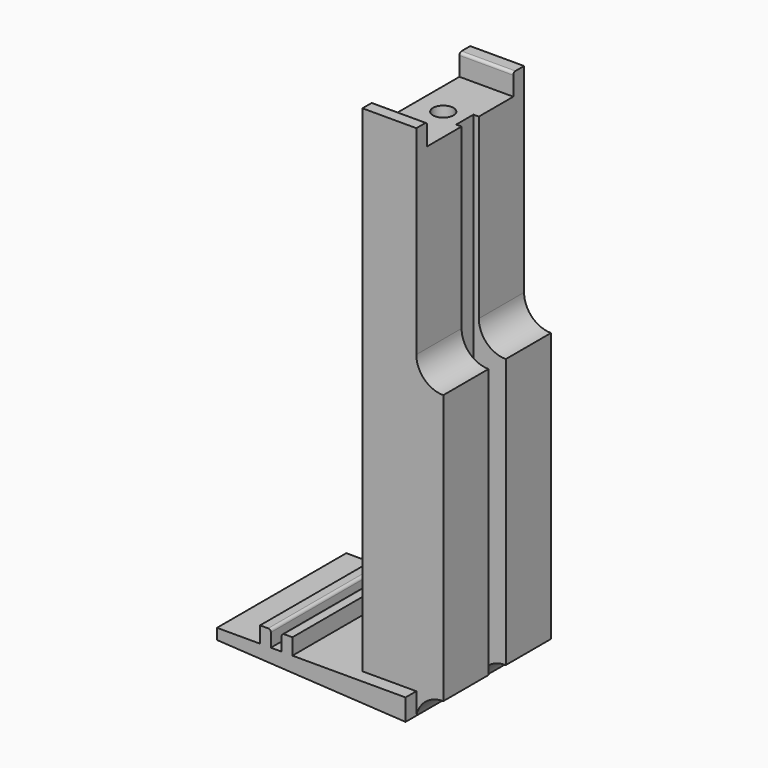
from build123d import *

# Parameters (mm, degrees)
F1_DEPTH      = 2
F2_R          = 1.9
F3_DEPTH      = 88
F4_W          = 2
F4_H          = 30
F5_DEPTH      = 3
F6_DEPTH      = 2
F8_DEPTH      = 30.001
F9_W          = 10
F9_H          = 2.5
F10_DEPTH     = 92
F11_R         = 0.5
F12_W         = 10.5
F12_H         = 50
F13_DEPTH     = 5
F14_T1_DEPTH  = 10.5
F14_T3_DEPTH  = 10.5
F14_T8_DEPTH  = 34.9948974279
F14_T13_DEPTH = 34.9948974279
F14_T18_DEPTH = 35.5
F14_T23_DEPTH = 35.5


# Not quite as in the source:
# - a fillet or chamfer that OpenCascade refuses, or shapes differently, is made with other operations: its cross-section is extruded or revolved along the edge and cut away or added


with BuildPart() as f1:
    # F0 (on Top) → F1 (new body)
    with BuildSketch(Plane.XY):
        Polygon((0, 2), (0, 15), (-35, 15), (-35, -15), (0, -15), (0, -2), (-1, -2), (-1, 2), align=None)
    extrude(amount=F1_DEPTH)

    # F2 (on face) → F3 (join)
    with BuildSketch(Plane.XY.offset(2)):
        Polygon((-1, 2), (0, 2), (0, 10), (-10, 10), (-10, -10), (0, -10), (0, -2), (-1, -2), align=None)
        with Locations((-5, 0)):
            Circle(F2_R, mode=Mode.SUBTRACT)
    extrude(amount=F3_DEPTH)

    # F4 (on face) → F5 (join)
    with BuildSketch(Plane.XY.offset(2)):
        with Locations((-26, 0)):
            Rectangle(F4_W, F4_H)
        with Locations((-22, 0)):
            Rectangle(F4_W, F4_H)
    extrude(amount=F5_DEPTH)

    # F6 (add): a face of the model
    f6_faces = [f1.faces().sort_by_distance(p)[0] for p in [
        (-17.5650095602, 0, 0),
    ]]
    extrude(f6_faces, amount=F6_DEPTH)

    # F7 (on face) → F8 (cut, through all)
    with BuildSketch(Plane.XZ.offset(15)):
        Polygon((0, -2), (-35, 0), (-35, -2), align=None)
    extrude(amount=-F8_DEPTH, mode=Mode.SUBTRACT)

    # F9 (on face) → F10 (join)
    with BuildSketch(Plane.XY.offset(2)):
        with Locations((-5, 11.25)):
            Rectangle(F9_W, F9_H)
        with Locations((-5, -11.25)):
            Rectangle(F9_W, F9_H)
    extrude(amount=F10_DEPTH)

    # F11
    f11_edges = [f1.edges().sort_by_distance(p)[0] for p in [
        (-25, 0, 5),
        (-23, 0, 5),
        (-5, 10, 94),
        (-5, -10, 94),
    ]]
    fillet(f11_edges, radius=F11_R)

    # F12 (on face) → F13 (join)
    with BuildSketch(Plane.YZ):
        with Locations((7.25, 27)):
            Rectangle(F12_W, F12_H)
        with Locations((-7.25, 27)):
            Rectangle(F12_W, F12_H)
    extrude(amount=F13_DEPTH)

    # F14: fillet of radius 5 on 4 edges, made by hand

    # F14_s2 → F14_t1 (join)
    with BuildSketch(Plane.XZ.offset(2)):
        with BuildLine():
            ThreePointArc((0, -2), (1.7367018254, 0.8729833462), (4.8989794856, 2))
            Line((4.8989794856, 2), (0, 2))
            Line((0, 2), (0, -2))
        make_face()
        with BuildLine():
            ThreePointArc((0, 57), (1.4644660941, 53.4644660941), (5, 52))
            Line((5, 52), (0, 52))
            Line((0, 52), (0, 57))
        make_face()
    extrude(amount=F14_T1_DEPTH)

    # F14_s4 → F14_t3 (join)
    with BuildSketch(Plane.XZ.offset(-12.5)):
        with BuildLine():
            ThreePointArc((0, -2), (1.7367018254, 0.8729833462), (4.8989794856, 2))
            Line((4.8989794856, 2), (0, 2))
            Line((0, 2), (0, -2))
        make_face()
        with BuildLine():
            ThreePointArc((0, 57), (1.4644660941, 53.4644660941), (5, 52))
            Line((5, 52), (0, 52))
            Line((0, 52), (0, 57))
        make_face()
    extrude(amount=F14_T3_DEPTH)


with BuildPart() as f14_tool6:
    # F14_s7 → F14_t8 (new body)
    with BuildSketch(Plane.XZ.offset(24.7474487139)):
        with BuildLine():
            ThreePointArc((0, -2), (1.7367018254, 0.8729833462), (4.8989794856, 2))
            Line((4.8989794856, 2), (0, 2))
            Line((0, 2), (0, -2))
        make_face()
    extrude(amount=-F14_T8_DEPTH)

    split(bisect_by=Plane.XZ.offset(-2), keep=Keep.BOTTOM)


with BuildPart() as f1_1:
    add(f1.part)

    # F14_t5: union F14_tool6
    add(f14_tool6.part)


with BuildPart() as f14_tool11:
    # F14_s12 → F14_t13 (new body)
    with BuildSketch(Plane.XZ.offset(10.2474487139)):
        with BuildLine():
            ThreePointArc((0, -2), (1.7367018254, 0.8729833462), (4.8989794856, 2))
            Line((4.8989794856, 2), (0, 2))
            Line((0, 2), (0, -2))
        make_face()
    extrude(amount=-F14_T13_DEPTH)

    split(bisect_by=Plane.XZ.offset(2), keep=Keep.TOP)


with BuildPart() as f1_2:
    add(f1_1.part)

    # F14_t10: union F14_tool11
    add(f14_tool11.part)


with BuildPart() as f14_tool16:
    # F14_s17 → F14_t18 (new body)
    with BuildSketch(Plane.XZ.offset(-10.5)):
        with BuildLine():
            ThreePointArc((0, 57), (1.4644660941, 53.4644660941), (5, 52))
            Line((5, 52), (0, 52))
            Line((0, 52), (0, 57))
        make_face()
    extrude(amount=F14_T18_DEPTH)

    split(bisect_by=Plane.XZ.offset(-2), keep=Keep.BOTTOM)


with BuildPart() as f1_3:
    add(f1_2.part)

    # F14_t15: union F14_tool16
    add(f14_tool16.part)


with BuildPart() as f14_tool21:
    # F14_s22 → F14_t23 (new body)
    with BuildSketch(Plane.XZ.offset(-25)):
        with BuildLine():
            ThreePointArc((0, 57), (1.4644660941, 53.4644660941), (5, 52))
            Line((5, 52), (0, 52))
            Line((0, 52), (0, 57))
        make_face()
    extrude(amount=F14_T23_DEPTH)

    split(bisect_by=Plane.XZ.offset(2), keep=Keep.TOP)


with BuildPart() as f1_4:
    add(f1_3.part)

    # F14_t20: union F14_tool21
    add(f14_tool21.part)


solid = f1_4.part
